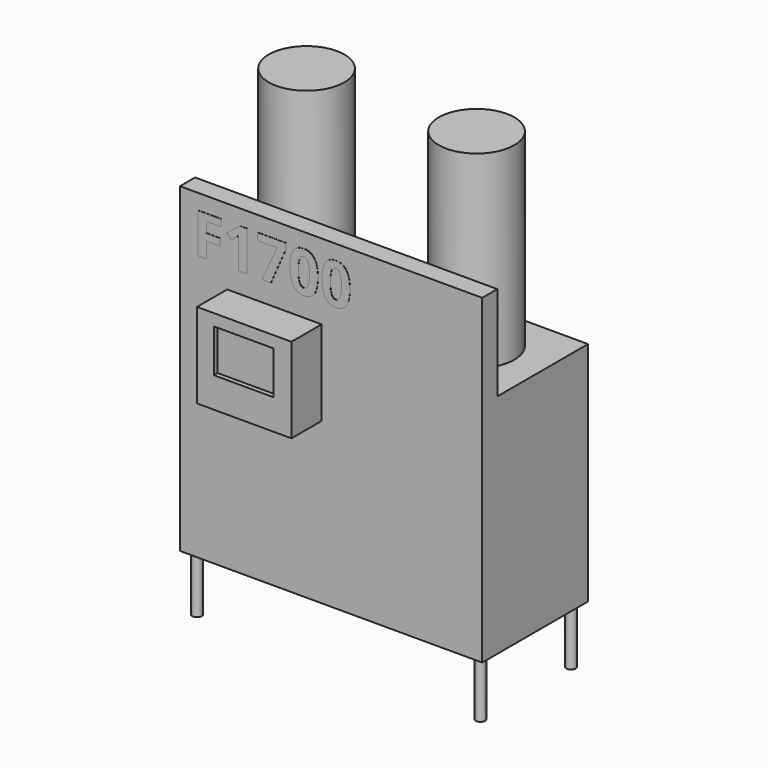
from build123d import *

# Parameters (mm, degrees)
F0_W          = 1600
F0_H          = 1700
F1_DEPTH      = 100
F2_W          = 500
F2_H          = 450
F3_DEPTH      = 200
F4_W          = 1600
F4_H          = 1200
F5_DEPTH      = 600
F6_R          = 200
F7_DEPTH      = 1000
F8_R          = 25
F9_DEPTH      = 300
F10_W         = 315.3864443302
F10_H         = 227.5288105011
F11_DEPTH     = 25
F12_TEXT_SIZE = 297.0884243647
F13_DEPTH     = 1


# Not quite as in the source:
# - Text() gives the source's letters only with a copy of the font that has no kerning and outlines rounded to 1/6400 em; it was checked with that copy


with BuildPart() as f1:
    # F0 (on Front) → F1 (new body)
    with BuildSketch(Plane.XZ):
        with Locations((800, 850)):
            Rectangle(F0_W, F0_H)
    extrude(amount=F1_DEPTH)

    # F2 (on face) → F3 (join)
    with BuildSketch(Plane.XZ.offset(100)):
        with Locations((500, 1075)):
            Rectangle(F2_W, F2_H)
    extrude(amount=F3_DEPTH)

    # F4 (on face) → F5 (join)
    with BuildSketch(Plane(origin=(0, 0, 0), x_dir=(-1, 0, 0), z_dir=(0, 1, 0))):
        with Locations((-800, 600)):
            Rectangle(F4_W, F4_H)
    extrude(amount=F5_DEPTH)

    # F6 (on face) → F7 (join)
    with BuildSketch(Plane.XY.offset(1200)):
        with Locations((350, 300)):
            Circle(F6_R)
        with Locations((1250, 300)):
            Circle(F6_R)
    extrude(amount=F7_DEPTH)

    # F8 (on face) → F9 (join)
    with BuildSketch(Plane(origin=(0, 0, 0), x_dir=(1, 0, 0), z_dir=(0, 0, -1))):
        with Locations((50, 50)):
            Circle(F8_R)
        with Locations((1550, 50)):
            Circle(F8_R)
        with Locations((50, -550)):
            Circle(F8_R)
        with Locations((1550, -550)):
            Circle(F8_R)
    extrude(amount=F9_DEPTH)

    # F10 (on face) → F11 (cut)
    with BuildSketch(Plane.XZ.offset(300)):
        with Locations((497.0036000013, 1124.523639679)):
            Rectangle(F10_W, F10_H)
    extrude(amount=-F11_DEPTH, mode=Mode.SUBTRACT)

    # F12 (on face) → F13 (join)
    with BuildSketch(Plane.XZ.offset(100)):
        with Locations((69.698870182, 1406.7474603653)):
            Text('F1700', F12_TEXT_SIZE, font='Open Sans', font_style=FontStyle.BOLD, text_align=(TextAlign.LEFT, TextAlign.BOTTOM))
    extrude(amount=F13_DEPTH)


solid = f1.part
